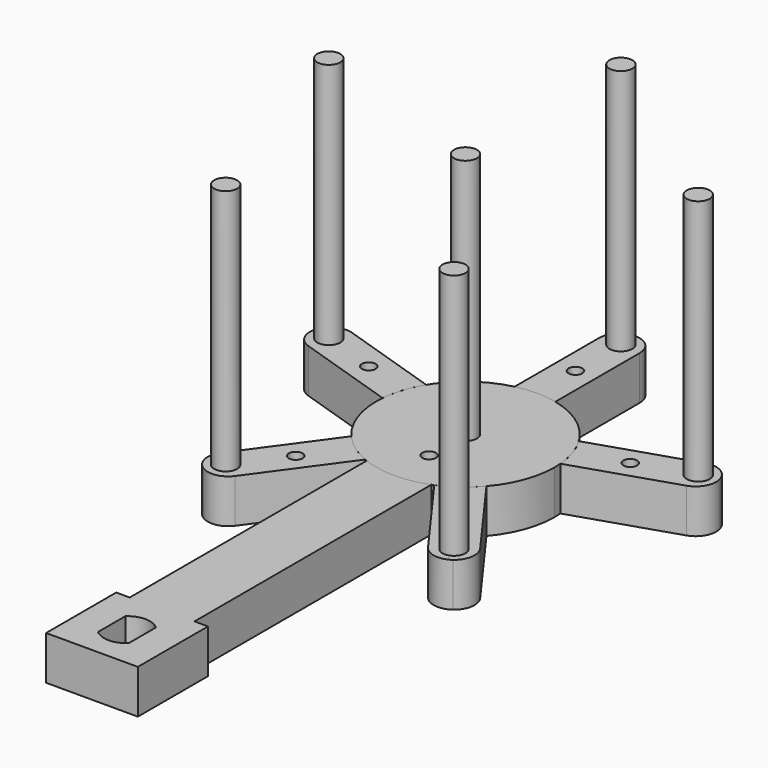
from build123d import *

# Parameters (mm, degrees)
F0_R     = 2.25
F0_R_2   = 1.35
F1_DEPTH = 8.6
F2_DEPTH = 8.6
F3_DEPTH = 57
F4_DEPTH = 8.6
F5_DEPTH = 57
F6_COUNT = 5
F7_R     = 3.99999
F7_2_R   = 3.99999
F7_3_R   = 3.99999
F7_4_R   = 3.99999
F7_5_R   = 3.99999


# Not quite as in the source:
# - a fillet or chamfer is up to 0.001 mm smaller than in the source, because OpenCascade refuses the exact size


with BuildPart() as f1:
    # F0 (on Top) → F1 (new body)
    with BuildSketch(Plane.XY):
        with BuildLine():
            ThreePointArc((6.35, -16.3099201064), (14.4477782812, -9.8791546507), (17.5024567955, 0))
            ThreePointArc((17.5024567955, 0), (13.7176131499, 10.8702844189), (4, 17.0392486301))
            ThreePointArc((4, 17.0392486301), (0, 17.5024567955), (-4, 17.0392486301))
            ThreePointArc((-4, 17.0392486301), (-17.4591634637, 1.2302865617), (-6.35, -16.3099201064))
            ThreePointArc((-6.35, -16.3099201064), (0, -17.5024567955), (6.35, -16.3099201064))
        make_face()
        with Locations((-0.0144804771, 0.0123086946)):
            Circle(F0_R, mode=Mode.SUBTRACT)
        with Locations((0, -8.9395707473)):
            Circle(F0_R_2, mode=Mode.SUBTRACT)
    extrude(amount=F1_DEPTH)

    # F0 (on Top) → F5 (join)
    with BuildSketch(Plane.XY):
        with Locations((-0.0144804771, 0.0123086946)):
            Circle(F0_R)
    extrude(amount=F5_DEPTH)


with BuildPart() as f2:
    # F0 (on Top) → F2 (new body)
    with BuildSketch(Plane.XY):
        with BuildLine():
            Line((6.35, -74.4), (6.35, -16.3099201064))
            ThreePointArc((6.35, -16.3099201064), (0, -17.5024567955), (-6.35, -16.3099201064))
            Line((-6.35, -16.3099201064), (-6.35, -74.4))
            Line((-6.35, -74.4), (0, -74.4))
            Line((0, -74.4), (6.35, -74.4))
        make_face()
        Polygon((9, -74.4), (6.35, -74.4), (0, -74.4), (-6.35, -74.4), (-9, -74.4), (-9, -91.6), (9, -91.6), align=None)
        with BuildLine():
            Line((3, -79.6458980338), (3, -86.3541019662))
            ThreePointArc((3, -86.3541019662), (0, -87.5), (-3, -86.3541019662))
            Line((-3, -86.3541019662), (-3, -79.6458980338))
            ThreePointArc((-3, -79.6458980338), (0, -78.5), (3, -79.6458980338))
        make_face(mode=Mode.SUBTRACT)
    extrude(amount=F2_DEPTH)


with BuildPart() as f3:
    # F0 (on Top) → F3 (new body)
    with BuildSketch(Plane.XY):
        with Locations((0, 38.1)):
            Circle(F0_R)
    extrude(amount=F3_DEPTH)


with BuildPart() as f4:
    # F0 (on Top) → F4 (new body)
    with BuildSketch(Plane.XY):
        with BuildLine():
            ThreePointArc((-4, 17.0392486301), (0, 17.5024567955), (4, 17.0392486301))
            Line((4, 17.0392486301), (4, 41.7012609541))
            Line((4, 41.7012609541), (0, 41.7012609541))
            Line((0, 41.7012609541), (-4, 41.7012609541))
            Line((-4, 41.7012609541), (-4, 17.0392486301))
        make_face()
        with Locations((0, 26.9654728472)):
            Circle(F0_R_2, mode=Mode.SUBTRACT)
        with Locations((0, 38.1)):
            Circle(F0_R, mode=Mode.SUBTRACT)
    extrude(amount=F4_DEPTH)


with BuildPart() as f6_1:
    # F6: instance of F4
    add(f4.part.rotate(Axis((0, 0, 0), (0, 0, 1)), 1 * 360 / F6_COUNT))

    # F7#2 (radius 4 in the source; OpenCascade refuses exactly that, so slightly less here)
    f7_2_edges = [f6_1.edges().sort_by_distance(p)[0] for p in [
        (-38.424188, 16.690624, 4.3),
        (-40.896324, 9.082172, 4.3),
    ]]
    fillet(f7_2_edges, radius=F7_2_R)


with BuildPart() as f6_2:
    # F6: instance of F4
    add(f4.part.rotate(Axis((0, 0, 0), (0, 0, 1)), 2 * 360 / F6_COUNT))

    # F7#3 (radius 4 in the source; OpenCascade refuses exactly that, so slightly less here)
    f7_3_edges = [f6_2.edges().sort_by_distance(p)[0] for p in [
        (-27.747454, -31.385888, 4.3),
        (-21.275318, -36.08817, 4.3),
    ]]
    fillet(f7_3_edges, radius=F7_3_R)


with BuildPart() as f6_3:
    # F6: instance of F4
    add(f4.part.rotate(Axis((0, 0, 0), (0, 0, 1)), 3 * 360 / F6_COUNT))

    # F7#4 (radius 4 in the source; OpenCascade refuses exactly that, so slightly less here)
    f7_4_edges = [f6_3.edges().sort_by_distance(p)[0] for p in [
        (27.747454, -31.385888, 4.3),
        (21.275318, -36.08817, 4.3),
    ]]
    fillet(f7_4_edges, radius=F7_4_R)


with BuildPart() as f6_4:
    # F6: instance of F4
    add(f4.part.rotate(Axis((0, 0, 0), (0, 0, 1)), 4 * 360 / F6_COUNT))

    # F7#5 (radius 4 in the source; OpenCascade refuses exactly that, so slightly less here)
    f7_5_edges = [f6_4.edges().sort_by_distance(p)[0] for p in [
        (38.424188, 16.690624, 4.3),
        (40.896324, 9.082172, 4.3),
    ]]
    fillet(f7_5_edges, radius=F7_5_R)


with BuildPart() as f6_5:
    # F6: instance of F3
    add(f3.part.rotate(Axis((0, 0, 0), (0, 0, 1)), 1 * 360 / F6_COUNT))


with BuildPart() as f6_6:
    # F6: instance of F3
    add(f3.part.rotate(Axis((0, 0, 0), (0, 0, 1)), 2 * 360 / F6_COUNT))


with BuildPart() as f6_7:
    # F6: instance of F3
    add(f3.part.rotate(Axis((0, 0, 0), (0, 0, 1)), 3 * 360 / F6_COUNT))


with BuildPart() as f6_8:
    # F6: instance of F3
    add(f3.part.rotate(Axis((0, 0, 0), (0, 0, 1)), 4 * 360 / F6_COUNT))


with BuildPart() as f4_1:
    add(f4.part)

    # F7 (radius 4 in the source; OpenCascade refuses exactly that, so slightly less here)
    f7_edges = [f4_1.edges().sort_by_distance(p)[0] for p in [
        (-4, 41.701261, 4.3),
        (4, 41.701261, 4.3),
    ]]
    fillet(f7_edges, radius=F7_R)


solid = Compound([f1.part, f2.part, f3.part, f6_1.part, f6_2.part, f6_3.part, f6_4.part, f6_5.part, f6_6.part, f6_7.part, f6_8.part, f4_1.part])
